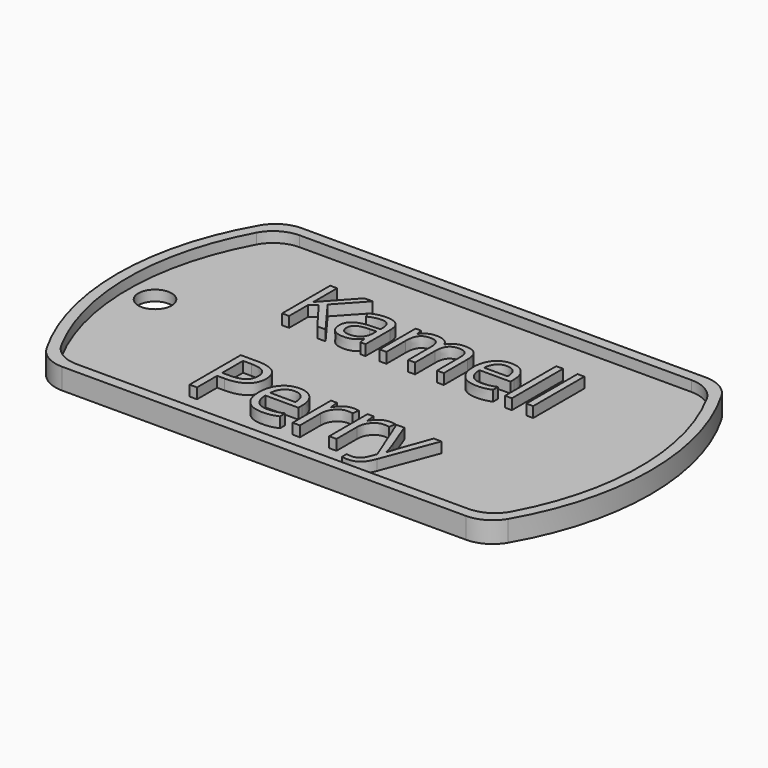
from build123d import *

# Parameters (mm, degrees)
F1_DEPTH     = 1
F3_DEPTH     = 1
F4_R         = 1.5875
F5_DEPTH     = 1
F6_TEXT_SIZE = 8.0192791453
F8_DEPTH     = 1
F7_TEXT_SIZE = 8.5327308625
F9_DEPTH     = 1


# Not quite as in the source:
# - Text() gives the source's letters only with a copy of the font that has no kerning and outlines rounded to 1/6400 em; it was checked with that copy


with BuildPart() as f1:
    # F0 (on Top) → F1 (new body)
    with BuildSketch(Plane.XY):
        with BuildLine():
            ThreePointArc((-19.2474145991, 14.2875), (-20.8349145991, 13.862130657), (-21.9970452561, 12.7))
            ThreePointArc((-21.9970452561, 12.7), (-25.4, 0), (-21.9970452561, -12.7))
            ThreePointArc((-21.9970452561, -12.7), (-20.8349145991, -13.862130657), (-19.2474145991, -14.2875))
            Line((-19.2474145991, -14.2875), (19.2474145991, -14.2875))
            ThreePointArc((19.2474145991, -14.2875), (20.8349145991, -13.862130657), (21.9970452561, -12.7))
            ThreePointArc((21.9970452561, -12.7), (25.4, 0), (21.9970452561, 12.7))
            ThreePointArc((21.9970452561, 12.7), (20.8349145991, 13.862130657), (19.2474145991, 14.2875))
            Line((19.2474145991, 14.2875), (-19.2474145991, 14.2875))
        make_face()
    extrude(amount=F1_DEPTH)

    # F2 (on face) → F3 (join)
    with BuildSketch(Plane.XY.offset(1)):
        with BuildLine():
            Line((19.2474145991, 14.2875), (-19.2474145991, 14.2875))
            ThreePointArc((-19.2474145991, 14.2875), (-20.8349145991, 13.862130657), (-21.9970452561, 12.7))
            ThreePointArc((-21.9970452561, 12.7), (-25.4, 0), (-21.9970452561, -12.7))
            ThreePointArc((-21.9970452561, -12.7), (-20.8349145991, -13.862130657), (-19.2474145991, -14.2875))
            Line((-19.2474145991, -14.2875), (19.2474145991, -14.2875))
            ThreePointArc((19.2474145991, -14.2875), (20.8349145991, -13.862130657), (21.9970452561, -12.7))
            ThreePointArc((21.9970452561, -12.7), (25.4, 0), (21.9970452561, 12.7))
            ThreePointArc((21.9970452561, 12.7), (20.8349145991, 13.862130657), (19.2474145991, 14.2875))
        make_face()
        with BuildLine():
            ThreePointArc((-21.4526124879, 11.6252061249), (-20.2856017842, 12.8404540819), (-18.6611352482, 13.2875))
            Line((-18.6611352482, 13.2875), (18.6611352482, 13.2875))
            ThreePointArc((18.6611352482, 13.2875), (20.2856017842, 12.8404540819), (21.4526124879, 11.6252061249))
            ThreePointArc((21.4526124879, 11.6252061249), (24.4, 0), (21.4526124879, -11.6252061249))
            ThreePointArc((21.4526124879, -11.6252061249), (20.2856017842, -12.8404540819), (18.6611352482, -13.2875))
            Line((18.6611352482, -13.2875), (-18.6611352482, -13.2875))
            ThreePointArc((-18.6611352482, -13.2875), (-20.2856017842, -12.8404540819), (-21.4526124879, -11.6252061249))
            ThreePointArc((-21.4526124879, -11.6252061249), (-24.4, 0), (-21.4526124879, 11.6252061249))
        make_face(mode=Mode.SUBTRACT)
    extrude(amount=F3_DEPTH)

    # F4 (on face) → F5 (cut)
    with BuildSketch(Plane.XY.offset(1)):
        with Locations((-21.821282804, 0)):
            Circle(F4_R)
    extrude(amount=-F5_DEPTH, mode=Mode.SUBTRACT)

    # F6 (on face) → F8 (join)
    with BuildSketch(Plane.XY.offset(1)):
        with Locations((-12.6140754931, 2.6512297336)):
            Text('Kamell', F6_TEXT_SIZE, font='Open Sans', text_align=(TextAlign.LEFT, TextAlign.BOTTOM))
    extrude(amount=F8_DEPTH)

    # F7 (on face) → F9 (join)
    with BuildSketch(Plane.XY.offset(1)):
        with Locations((-10.8685659361, -10.618503904)):
            Text('Perry', F7_TEXT_SIZE, font='Open Sans', text_align=(TextAlign.LEFT, TextAlign.BOTTOM))
    extrude(amount=F9_DEPTH)


solid = f1.part
